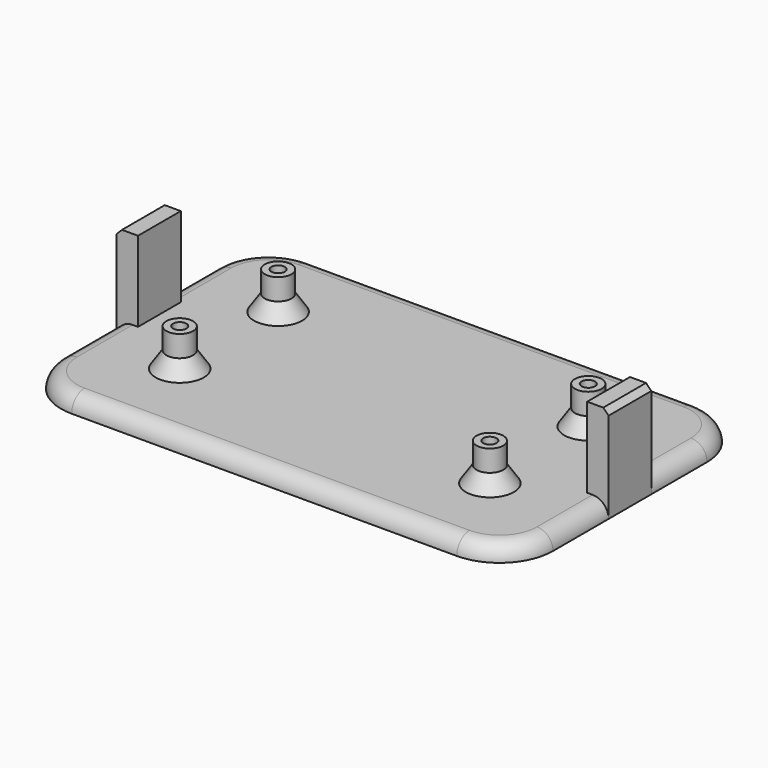
from build123d import *

# Parameters (mm, degrees)
F2_DEPTH = 3
F1_R     = 2.5
F1_R_2   = 1.25
F3_DEPTH = 10
F4_SIZE2 = 3
F4_SIZE  = 2
F5_R     = 2.99999
F7_W     = 10
F7_H     = 18
F8_DEPTH = 4
F10_SIZE = 1


# Not quite as in the source:
# - a fillet or chamfer is up to 0.001 mm smaller than in the source, because OpenCascade refuses the exact size


with BuildPart() as f2:
    # F0 (on Top) → F2 (new body)
    with BuildSketch(Plane.XY):
        with BuildLine():
            ThreePointArc((46, 18), (43.0710678119, 25.0710678119), (36, 28))
            Line((36, 28), (-36, 28))
            ThreePointArc((-36, 28), (-43.0710678119, 25.0710678119), (-46, 18))
            Line((-46, 18), (-46, -18))
            ThreePointArc((-46, -18), (-43.0710678119, -25.0710678119), (-36, -28))
            Line((-36, -28), (36, -28))
            ThreePointArc((36, -28), (43.0710678119, -25.0710678119), (46, -18))
            Line((46, -18), (46, 18))
        make_face()
    extrude(amount=F2_DEPTH)

    # F1 (on Top) → F3 (join)
    with BuildSketch(Plane.XY):
        with Locations((-29, 11.5)):
            Circle(F1_R)
        with Locations((-29, 11.5)):
            Circle(F1_R_2, mode=Mode.SUBTRACT)
        with Locations((29, 11.5)):
            Circle(F1_R)
        with Locations((29, 11.5)):
            Circle(F1_R_2, mode=Mode.SUBTRACT)
        with Locations((-29, -11.5)):
            Circle(F1_R)
        with Locations((-29, -11.5)):
            Circle(F1_R_2, mode=Mode.SUBTRACT)
        with Locations((29, -11.5)):
            Circle(F1_R)
        with Locations((29, -11.5)):
            Circle(F1_R_2, mode=Mode.SUBTRACT)
    extrude(amount=F3_DEPTH)

    # F4
    f4_edges = [f2.edges().sort_by_distance(p)[0] for p in [
        (-31.5, 11.5, 3),
        (26.5, 11.5, 3),
        (26.5, -11.5, 3),
        (-31.5, -11.5, 3),
    ]]
    chamfer(f4_edges, length=F4_SIZE, length2=F4_SIZE2)

    # F5 (radius 3 in the source; OpenCascade refuses exactly that, so slightly less here)
    f5_edges = [f2.edges().sort_by_distance(p)[0] for p in [
        (0, 28, 3),
    ]]
    fillet(f5_edges, radius=F5_R)

    # F7 (on offset) → F8 (join)
    with BuildSketch(Plane.YZ.offset(46)):
        with Locations((0, 9)):
            Rectangle(F7_W, F7_H)
    extrude(amount=-F8_DEPTH)

    # F9: F2 across plane


with BuildPart() as f2_1:
    add(f2.part)
    add(f2.part.mirror(Plane.YZ))

    # F10
    f10_edges = [f2_1.edges().sort_by_distance(p)[0] for p in [
        (-46, 0, 18),
        (46, 0, 18),
    ]]
    chamfer(f10_edges, length=F10_SIZE)


solid = f2_1.part
